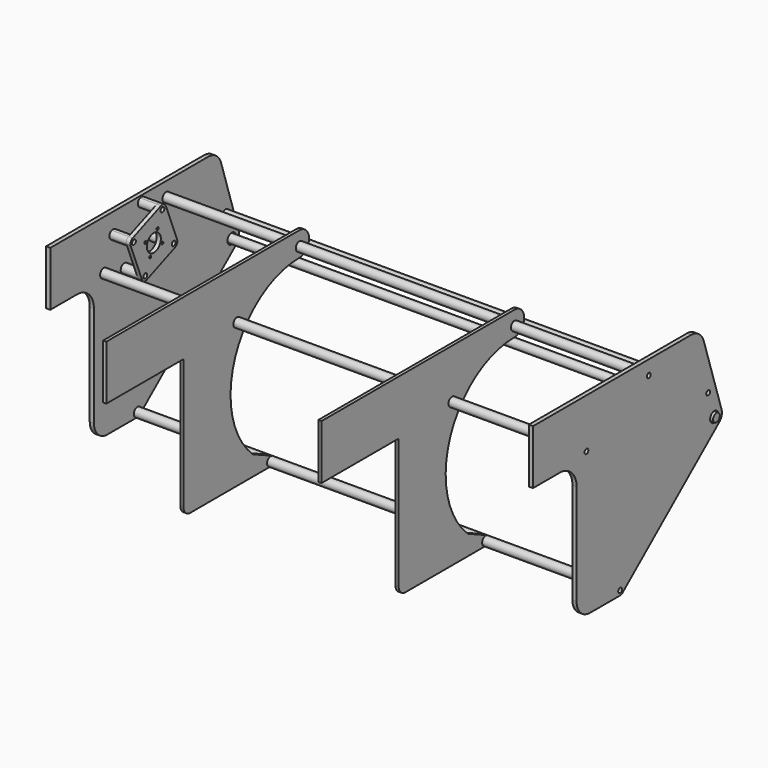
from build123d import *

# Parameters (mm, degrees)
F5_R           = 3.571875
F5_R_2         = 7.9375
F6_DEPTH       = 6.35
F7_R           = 3.571875
F8_DEPTH       = 4.7625
F9_R           = 6.858
F9_R_2         = 4.3688
F10_DEPTH      = 196.85
F12_DEPTH      = 196.85
F12_DEPTH_BACK = 527.05
F13_R          = 6.858
F13_R_2        = 4.3688
F14_DEPTH      = 320.675
F2_R           = 6.35
F15_DEPTH      = 371.475
F15_DEPTH_BACK = 371.475
F18_R          = 1.984375
F18_R_2        = 13.208
F18_R_3        = 3.571875
F19_DEPTH      = 6.35
F20_DEPTH      = 25.4


# Not quite as in the source:
# - a variable given as a bare number and used for a length is read in inches; the dataset says mm whatever the document's units were


with BuildPart() as f6:
    # F5 (on offset) → F6 (new body)
    with BuildSketch(Plane.YZ.offset(368.3)):
        with BuildLine():
            ThreePointArc((-173.8703164042, 71.0483314652), (-172.0552224643, 73.406227646), (-171.4096814604, 76.3109681202))
            ThreePointArc((-171.4096814604, 76.3109681202), (-183.1170197657, 81.1603064256), (-178.2676814604, 69.4529681202))
            ThreePointArc((-178.2676814604, 69.4529681202), (-175.9287712633, 69.8641345494), (-173.8703164042, 71.0483314652))
        make_face()
        with Locations((-178.2676814604, 76.3109681202)):
            Circle(F5_R, mode=Mode.SUBTRACT)
        with BuildLine():
            ThreePointArc((-178.2676814604, 69.4529681202), (-183.1170197657, 81.1603064256), (-171.4096814604, 76.3109681202))
            ThreePointArc((-171.4096814604, 76.3109681202), (-172.0552224643, 73.406227646), (-173.8703164042, 71.0483314652))
            Line((-173.8703164042, 71.0483314652), (9.1611772003, 223.9861736353))
            ThreePointArc((9.1611772003, 223.9861736353), (13.7228105902, 230.9729249747), (13.6040272642, 239.3161308325))
            Line((13.6040272642, 239.3161308325), (-20.0937695737, 344.3120103688))
            ThreePointArc((-20.0937695737, 344.3120103688), (-29.3119949247, 357.0721229819), (-44.2787069322, 361.95))
            Line((-44.2787069322, 361.95), (-343.0228039623, 361.95))
            Line((-343.0228039623, 361.95), (-343.0228039623, 279.4))
            Line((-343.0228039623, 279.4), (-292.2228039623, 279.4))
            ThreePointArc((-292.2228039623, 279.4), (-269.7721636596, 270.1006403027), (-260.4728039623, 247.65))
            Line((-260.4728039623, 247.65), (-260.4728039623, 94.8529681202))
            ThreePointArc((-260.4728039623, 94.8529681202), (-253.0333162044, 76.8924558781), (-235.0728039623, 69.4529681202))
            Line((-235.0728039623, 69.4529681202), (-178.2676814604, 69.4529681202))
        make_face()
        with Locations((-241.9780255837, 287.3045874986)):
            Circle(F5_R, mode=Mode.SUBTRACT)
        with Locations((0, 234.95)):
            Circle(F5_R_2, mode=Mode.SUBTRACT)
        with Locations((-11.7982557606, 271.7111047849)):
            Circle(F5_R, mode=Mode.SUBTRACT)
        with Locations((-123.9478039623, 340.4723484299)):
            Circle(F5_R, mode=Mode.SUBTRACT)
    extrude(amount=-F6_DEPTH)


with BuildPart() as f8:
    # F7 (on offset) → F8 (new body)
    with BuildSketch(Plane.YZ.offset(165.1)):
        with BuildLine():
            Line((-489.0728039623, 279.4), (-362.0728039623, 279.4))
            Line((-362.0728039623, 279.4), (-343.0228039623, 279.4))
            Line((-343.0228039623, 279.4), (-343.0228039623, 152.4))
            Line((-343.0228039623, 152.4), (-343.0228039623, 82.1529681202))
            ThreePointArc((-343.0228039623, 82.1529681202), (-339.3030600834, 73.1727119992), (-330.3228039623, 69.4529681202))
            Line((-330.3228039623, 69.4529681202), (-178.2676814604, 69.4529681202))
            ThreePointArc((-178.2676814604, 69.4529681202), (-171.566605749, 74.8522877882), (-175.4170756441, 82.5484524273))
            Line((-175.4170756441, 82.5484524273), (-211.9442187549, 99.2417988913))
            ThreePointArc((-211.9442187549, 99.2417988913), (-245.2592723877, 242.3826003236), (-123.9478039623, 325.3446968599))
            ThreePointArc((-123.9478039623, 325.3446968599), (-105.6451523922, 343.6473484299), (-123.9478039623, 361.95))
            Line((-123.9478039623, 361.95), (-362.0728039623, 361.95))
            Line((-362.0728039623, 361.95), (-489.0728039623, 361.95))
            Line((-489.0728039623, 361.95), (-489.0728039623, 279.4))
        make_face()
        with Locations((-178.2676814604, 76.3109681202)):
            Circle(F7_R, mode=Mode.SUBTRACT)
        with Locations((-241.9780255837, 287.3045874986)):
            Circle(F7_R, mode=Mode.SUBTRACT)
        with Locations((-123.9478039623, 340.4723484299)):
            Circle(F7_R, mode=Mode.SUBTRACT)
    extrude(amount=-F8_DEPTH)


with BuildPart() as f10:
    # F9 (on face) → F10 (new body, through all)
    with BuildSketch(Plane.YZ.offset(165.1)):
        with Locations((-123.9478039623, 340.4723484299)):
            Circle(F9_R)
        with Locations((-123.9478039623, 340.4723484299)):
            Circle(F9_R_2, mode=Mode.SUBTRACT)
    extrude(amount=F10_DEPTH)


with BuildPart() as f10b:
    # F9 (on face) → F10, piece 2 (new body, through all)
    with BuildSketch(Plane.YZ.offset(165.1)):
        with Locations((-241.9780255837, 287.3045874986)):
            Circle(F9_R)
        with Locations((-241.9780255837, 287.3045874986)):
            Circle(F9_R_2, mode=Mode.SUBTRACT)
    extrude(amount=F10_DEPTH)


with BuildPart() as f10c:
    # F9 (on face) → F10, piece 3 (new body, through all)
    with BuildSketch(Plane.YZ.offset(165.1)):
        with BuildLine():
            ThreePointArc((-178.2676814604, 69.4529681202), (-173.418343155, 71.4616298149), (-171.4096814604, 76.3109681202))
            ThreePointArc((-171.4096814604, 76.3109681202), (-172.4978626293, 80.0179014426), (-175.4170756441, 82.5484524273))
            ThreePointArc((-175.4170756441, 82.5484524273), (-184.9687571717, 77.7696484523), (-178.2676814604, 69.4529681202))
        make_face()
        with Locations((-178.2676814604, 76.3109681202)):
            Circle(F9_R_2, mode=Mode.SUBTRACT)
    extrude(amount=F10_DEPTH)


with BuildPart() as f11_1:
    # F11: instance of F8
    add(f8.part.mirror(Plane.YZ))


with BuildPart() as f11_2:
    # F11: instance of F6
    add(f6.part.mirror(Plane.YZ))


with BuildPart() as f11_3:
    # F11: instance of F10
    add(f10.part.mirror(Plane.YZ))


with BuildPart() as f11_4:
    # F11: instance of F10b
    add(f10b.part.mirror(Plane.YZ))


with BuildPart() as f11_5:
    # F11: instance of F10c
    add(f10c.part.mirror(Plane.YZ))


with BuildPart() as f12:
    # F9 (on face) → F12 (new body, two sides)
    with BuildSketch(Plane.YZ.offset(165.1)) as f12_sk:
        with Locations((-11.7982557606, 271.7111047849)):
            Circle(F9_R)
        with Locations((-11.7982557606, 271.7111047849)):
            Circle(F9_R_2, mode=Mode.SUBTRACT)
    extrude(amount=F12_DEPTH)
    extrude(f12_sk.sketch, amount=-F12_DEPTH_BACK)


with BuildPart() as f14:
    # F13 (on face) → F14 (new body, through all)
    with BuildSketch(Plane.YZ.offset(-160.3375)):
        with Locations((-241.9780255837, 287.3045874986)):
            Circle(F13_R)
        with Locations((-241.9780255837, 287.3045874986)):
            Circle(F13_R_2, mode=Mode.SUBTRACT)
    extrude(amount=F14_DEPTH)


with BuildPart() as f14b:
    # F13 (on face) → F14, piece 2 (new body, through all)
    with BuildSketch(Plane.YZ.offset(-160.3375)):
        with Locations((-123.9478039623, 340.4723484299)):
            Circle(F13_R)
        with Locations((-123.9478039623, 340.4723484299)):
            Circle(F13_R_2, mode=Mode.SUBTRACT)
    extrude(amount=F14_DEPTH)


with BuildPart() as f14c:
    # F13 (on face) → F14, piece 3 (new body, through all)
    with BuildSketch(Plane.YZ.offset(-160.3375)):
        with Locations((-178.2676814604, 76.3109681202)):
            Circle(F13_R)
        with Locations((-178.2676814604, 76.3109681202)):
            Circle(F13_R_2, mode=Mode.SUBTRACT)
    extrude(amount=F14_DEPTH)


with BuildPart() as f15:
    # F2 (on Right) → F15 (new body, two sides)
    with BuildSketch(Plane.YZ) as f15_sk:
        with Locations((0, 234.95)):
            Circle(F2_R)
    extrude(amount=F15_DEPTH)
    extrude(f15_sk.sketch, amount=-F15_DEPTH_BACK)


with BuildPart() as f19:
    # F18 (on offset) → F19 (new body)
    with BuildSketch(Plane.YZ.offset(-336.55)):
        with BuildLine():
            Line((-173.1817063766, 359.4184532821), (-226.8466327762, 338.103314647))
            ThreePointArc((-226.8466327762, 338.103314647), (-220.4634100199, 337.4038815178), (-217.4570860582, 331.7296630081))
            ThreePointArc((-217.4570860582, 331.7296630081), (-223.0263539177, 324.9938383763), (-230.6887376972, 329.1981162901))
            Line((-230.6887376972, 329.1981162901), (-209.3735990622, 275.5331898906))
            ThreePointArc((-209.3735990622, 275.5331898906), (-204.2886795637, 284.8005612403), (-196.1419474232, 278.0647366085))
            ThreePointArc((-196.1419474232, 278.0647366085), (-197.3257289135, 274.2130605702), (-200.4684007053, 271.6910849696))
            Line((-200.4684007053, 271.6910849696), (-146.8034743057, 293.0062236046))
            ThreePointArc((-146.8034743057, 293.0062236046), (-155.6319471696, 302.0966536872), (-142.9613693847, 301.9114219615))
            Line((-142.9613693847, 301.9114219615), (-164.2765080197, 355.576348361))
            ThreePointArc((-164.2765080197, 355.576348361), (-163.9143350269, 354.3335337836), (-163.7921596587, 353.0448016431))
            ThreePointArc((-163.7921596587, 353.0448016431), (-174.501835697, 347.3705831334), (-173.1817063766, 359.4184532821))
        make_face()
        with Locations((-193.7578696435, 299.4859464792)):
            Circle(F18_R, mode=Mode.SUBTRACT)
        with Locations((-202.8938761875, 322.4875852284)):
            Circle(F18_R, mode=Mode.SUBTRACT)
        with Locations((-186.8250535409, 315.5547691258)):
            Circle(F18_R_2, mode=Mode.SUBTRACT)
        with Locations((-170.7562308943, 308.6219530232)):
            Circle(F18_R, mode=Mode.SUBTRACT)
        with Locations((-179.8922374384, 331.6235917724)):
            Circle(F18_R, mode=Mode.SUBTRACT)
        with BuildLine():
            ThreePointArc((-164.2765080197, 355.576348361), (-167.933381215, 359.3417277891), (-173.1817063766, 359.4184532821))
            ThreePointArc((-173.1817063766, 359.4184532821), (-174.501835697, 347.3705831334), (-163.7921596587, 353.0448016431))
            ThreePointArc((-163.7921596587, 353.0448016431), (-163.9143350269, 354.3335337836), (-164.2765080197, 355.576348361))
        make_face()
        with Locations((-170.6501596587, 353.0448016431)):
            Circle(F18_R_3, mode=Mode.SUBTRACT)
        with BuildLine():
            ThreePointArc((-217.4570860582, 331.7296630081), (-220.4634100199, 337.4038815178), (-226.8466327762, 338.103314647))
            ThreePointArc((-226.8466327762, 338.103314647), (-230.6120122042, 334.4464414518), (-230.6887376972, 329.1981162901))
            ThreePointArc((-230.6887376972, 329.1981162901), (-223.0263539177, 324.9938383763), (-217.4570860582, 331.7296630081))
        make_face()
        with Locations((-224.3150860582, 331.7296630081)):
            Circle(F18_R_3, mode=Mode.SUBTRACT)
        with BuildLine():
            ThreePointArc((-142.4770210237, 299.3798752435), (-142.5991963919, 300.668607384), (-142.9613693847, 301.9114219615))
            ThreePointArc((-142.9613693847, 301.9114219615), (-155.6319471696, 302.0966536872), (-146.8034743057, 293.0062236046))
            ThreePointArc((-146.8034743057, 293.0062236046), (-143.6608025139, 295.5281992052), (-142.4770210237, 299.3798752435))
        make_face()
        with Locations((-149.3350210237, 299.3798752435)):
            Circle(F18_R_3, mode=Mode.SUBTRACT)
        with BuildLine():
            ThreePointArc((-196.1419474232, 278.0647366085), (-204.2886795637, 284.8005612403), (-209.3735990622, 275.5331898906))
            ThreePointArc((-209.3735990622, 275.5331898906), (-205.7167258669, 271.7678104625), (-200.4684007053, 271.6910849696))
            ThreePointArc((-200.4684007053, 271.6910849696), (-197.3257289135, 274.2130605702), (-196.1419474232, 278.0647366085))
        make_face()
        with Locations((-202.9999474232, 278.0647366085)):
            Circle(F18_R_3, mode=Mode.SUBTRACT)
    extrude(amount=F19_DEPTH)


with BuildPart() as f20:
    # F18 (on offset) → F20 (new body, through all)
    with BuildSketch(Plane.YZ.offset(-336.55)):
        with BuildLine():
            ThreePointArc((-164.2765080197, 355.576348361), (-167.933381215, 359.3417277891), (-173.1817063766, 359.4184532821))
            ThreePointArc((-173.1817063766, 359.4184532821), (-174.501835697, 347.3705831334), (-163.7921596587, 353.0448016431))
            ThreePointArc((-163.7921596587, 353.0448016431), (-163.9143350269, 354.3335337836), (-164.2765080197, 355.576348361))
        make_face()
        with Locations((-170.6501596587, 353.0448016431)):
            Circle(F18_R_3, mode=Mode.SUBTRACT)
    extrude(amount=-F20_DEPTH)


with BuildPart() as f20b:
    # F18 (on offset) → F20, piece 2 (new body, through all)
    with BuildSketch(Plane.YZ.offset(-336.55)):
        with BuildLine():
            ThreePointArc((-217.4570860582, 331.7296630081), (-220.4634100199, 337.4038815178), (-226.8466327762, 338.103314647))
            ThreePointArc((-226.8466327762, 338.103314647), (-230.6120122042, 334.4464414518), (-230.6887376972, 329.1981162901))
            ThreePointArc((-230.6887376972, 329.1981162901), (-223.0263539177, 324.9938383763), (-217.4570860582, 331.7296630081))
        make_face()
        with Locations((-224.3150860582, 331.7296630081)):
            Circle(F18_R_3, mode=Mode.SUBTRACT)
    extrude(amount=-F20_DEPTH)


with BuildPart() as f20c:
    # F18 (on offset) → F20, piece 3 (new body, through all)
    with BuildSketch(Plane.YZ.offset(-336.55)):
        with BuildLine():
            ThreePointArc((-142.4770210237, 299.3798752435), (-142.5991963919, 300.668607384), (-142.9613693847, 301.9114219615))
            ThreePointArc((-142.9613693847, 301.9114219615), (-155.6319471696, 302.0966536872), (-146.8034743057, 293.0062236046))
            ThreePointArc((-146.8034743057, 293.0062236046), (-143.6608025139, 295.5281992052), (-142.4770210237, 299.3798752435))
        make_face()
        with Locations((-149.3350210237, 299.3798752435)):
            Circle(F18_R_3, mode=Mode.SUBTRACT)
    extrude(amount=-F20_DEPTH)


with BuildPart() as f20d:
    # F18 (on offset) → F20, piece 4 (new body, through all)
    with BuildSketch(Plane.YZ.offset(-336.55)):
        with BuildLine():
            ThreePointArc((-196.1419474232, 278.0647366085), (-204.2886795637, 284.8005612403), (-209.3735990622, 275.5331898906))
            ThreePointArc((-209.3735990622, 275.5331898906), (-205.7167258669, 271.7678104625), (-200.4684007053, 271.6910849696))
            ThreePointArc((-200.4684007053, 271.6910849696), (-197.3257289135, 274.2130605702), (-196.1419474232, 278.0647366085))
        make_face()
        with Locations((-202.9999474232, 278.0647366085)):
            Circle(F18_R_3, mode=Mode.SUBTRACT)
    extrude(amount=-F20_DEPTH)


solid = Compound([f6.part, f8.part, f10.part, f10b.part, f10c.part, f11_1.part, f11_2.part, f11_3.part, f11_4.part, f11_5.part, f12.part, f14.part, f14b.part, f14c.part, f15.part, f19.part, f20.part, f20b.part, f20c.part, f20d.part])
